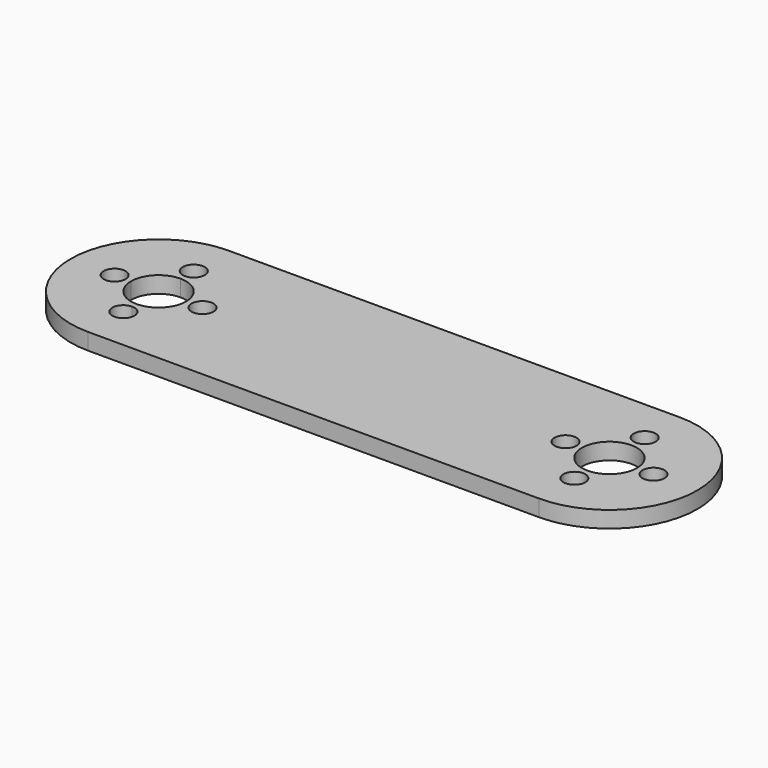
from build123d import *

# Parameters (mm, degrees)
F0_R     = 1.5875
F1_DEPTH = 2.38125


# Not quite as in the source:
# - a length typed as a fraction of an inch, garbled in the dataset ("3 / 203.2 mm" for 3/8 in), is restored


with BuildPart() as f1:
    # F0 (on Top) → F1 (new body)
    with BuildSketch(Plane.XY):
        with BuildLine():
            Line((0, -12.7), (0, 0))
            Line((0, 0), (0, 12.7))
            Line((0, 12.7), (-32.55645, 12.7))
            ThreePointArc((-32.55645, 12.7), (-45.25645, 0), (-32.55645, -12.7))
            Line((-32.55645, -12.7), (0, -12.7))
        make_face()
        with BuildLine():
            ThreePointArc((-30.96895, -6.35), (-33.6789820151, -7.4725320151), (-32.55645, -4.7625))
            ThreePointArc((-32.55645, -4.7625), (-31.4339179849, -5.2274679849), (-30.96895, -6.35))
        make_face(mode=Mode.SUBTRACT)
        with Locations((-38.90645, 0)):
            Circle(F0_R, mode=Mode.SUBTRACT)
        with BuildLine():
            ThreePointArc((-32.55645, 3.96875), (-29.7501199622, 2.8063300378), (-28.5877, 0))
            ThreePointArc((-28.5877, 0), (-29.7501199622, -2.8063300378), (-32.55645, -3.96875))
            ThreePointArc((-32.55645, -3.96875), (-35.3627800378, -2.8063300378), (-36.5252, 0))
            ThreePointArc((-36.5252, 0), (-35.3627800378, 2.8063300378), (-32.55645, 3.96875))
        make_face(mode=Mode.SUBTRACT)
        with BuildLine():
            ThreePointArc((-24.61895, 0), (-26.20645, -1.5875), (-27.79395, 0))
            ThreePointArc((-27.79395, 0), (-26.20645, 1.5875), (-24.61895, 0))
        make_face(mode=Mode.SUBTRACT)
        with BuildLine():
            ThreePointArc((-30.96895, 6.35), (-31.4339179849, 5.2274679849), (-32.55645, 4.7625))
            ThreePointArc((-32.55645, 4.7625), (-33.6789820151, 7.4725320151), (-30.96895, 6.35))
        make_face(mode=Mode.SUBTRACT)
        with BuildLine():
            Line((0, 12.7), (0, 0))
            Line((0, 0), (0, -12.7))
            Line((0, -12.7), (32.54375, -12.7))
            ThreePointArc((32.54375, -12.7), (45.24375, 0), (32.54375, 12.7))
            Line((32.54375, 12.7), (0, 12.7))
        make_face()
        with Locations((32.55645, -6.35)):
            Circle(F0_R, mode=Mode.SUBTRACT)
        with BuildLine():
            ThreePointArc((27.79395, 0), (26.20645, -1.5875), (24.61895, 0))
            ThreePointArc((24.61895, 0), (26.20645, 1.5875), (27.79395, 0))
        make_face(mode=Mode.SUBTRACT)
        with BuildLine():
            ThreePointArc((36.5125, 0), (32.54375, -3.96875), (28.575, 0))
            ThreePointArc((28.575, 0), (32.54375, 3.96875), (36.5125, 0))
        make_face(mode=Mode.SUBTRACT)
        with Locations((38.90645, 0)):
            Circle(F0_R, mode=Mode.SUBTRACT)
        with Locations((32.55645, 6.35)):
            Circle(F0_R, mode=Mode.SUBTRACT)
    extrude(amount=F1_DEPTH)


solid = f1.part
